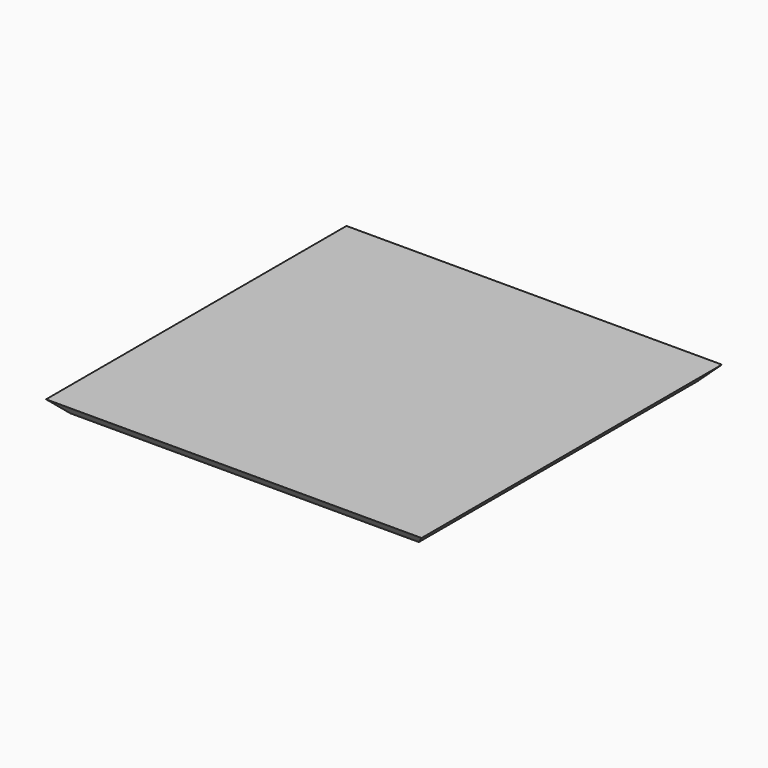
from build123d import *

# Parameters (mm, degrees)
F0_W     = 533.4
F0_H     = 533.4
F1_DEPTH = 19.05
F2_SIZE  = 19.04999


# Not quite as in the source:
# - a fillet or chamfer is up to 0.001 mm smaller than in the source, because OpenCascade refuses the exact size


with BuildPart() as f1:
    # F0 (on Top) → F1 (new body)
    with BuildSketch(Plane.XY):
        with Locations((8.2681225613, 47.9035311963)):
            Rectangle(F0_W, F0_H)
    extrude(amount=F1_DEPTH)

    # F2 (size 19.05 in the source; OpenCascade refuses exactly that, so slightly less here)
    f2_edges = [f1.edges().sort_by_distance(p)[0] for p in [
        (-258.431877, 47.903531, 0),
        (8.268123, -218.796469, 0),
        (274.968123, 47.903531, 0),
        (8.268123, 314.603531, 0),
    ]]
    chamfer(f2_edges, length=F2_SIZE)


solid = f1.part
